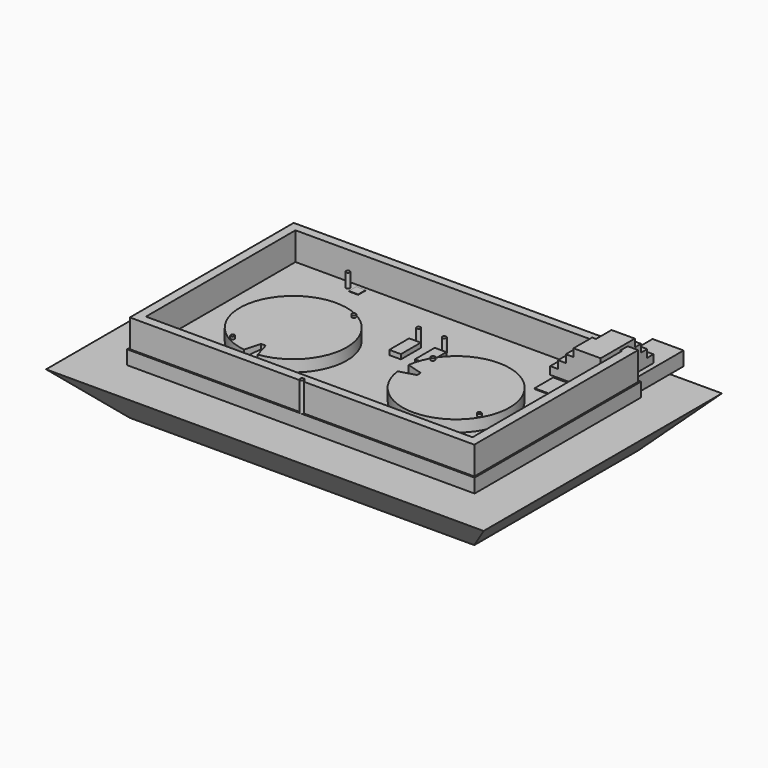
from build123d import *

# Parameters (mm, degrees)
F0_W        = 11277.6
F0_H        = 6705.6
F1_DEPTH    = 457.2
F2_W        = 11277.6
F2_H        = 6705.6
F2_W_2      = 10668
F2_H_2      = 6096
F3_DEPTH    = 914.4
F4_R        = 1752.6
F5_DEPTH    = 381
F6_W        = 304.8
F6_H        = 304.8
F7_DEPTH    = 12.7
F8_W        = 381
F8_H        = 812.8
F9_DEPTH    = 152.4
F11_W       = 11277.6
F11_H       = 6705.6
F12_DEPTH   = 1524
F12_TAPER   = -45
F14_R       = 63.5
F15_DEPTH   = 457.2
F16_DEPTH   = 508
F17_W       = 10693.4
F17_H       = 6121.4
F17_W_2     = 10668
F17_H_2     = 6096
F18_DEPTH   = 914.4
F21_DEPTH   = 228.6
F22_SIZE2   = 533.39999
F22_SIZE    = 76.19999
F22_2_SIZE2 = 533.39999
F22_2_SIZE  = 76.19999
F23_W       = 11379.2
F23_H       = 6807.2
F23_W_2     = 11277.6
F23_H_2     = 6705.6
F24_DEPTH   = 457.2
F25_W       = 1016
F25_H       = 457.2
F26_DEPTH   = 2032
F27_R       = 25.4
F28_DEPTH   = 1816.1010001
F30_DEPTH   = 1016
F32_DEPTH   = 762
F34_DEPTH   = 762
F36_DEPTH   = 25.4


# Not quite as in the source:
# - a fillet or chamfer is up to 0.001 mm smaller than in the source, because OpenCascade refuses the exact size


with BuildPart() as f1:
    # F0 (on Top) → F1 (new body)
    with BuildSketch(Plane.XY):
        Rectangle(F0_W, F0_H)
    extrude(amount=-F1_DEPTH)

    # F23 (on Top) → F24 (join, through all)
    with BuildSketch(Plane.XY):
        Rectangle(F23_W, F23_H)
        Rectangle(F23_W_2, F23_H_2, mode=Mode.SUBTRACT)
    extrude(amount=-F24_DEPTH)

    # F25 (on face) → F26 (join)
    with BuildSketch(Plane(origin=(0, 3403.6, 0), x_dir=(-1, 0, 0), z_dir=(0, 1, 0))):
        with Locations((-4953, -228.6)):
            Rectangle(F25_W, F25_H)
    extrude(amount=F26_DEPTH)

    # F35 (on face) → F36 (join)
    with BuildSketch(Plane.XY):
        with BuildLine():
            Line((5041.9, 2146.3), (3822.7, 2146.3))
            Line((3822.7, 2146.3), (3822.7, 1384.3))
            Line((3822.7, 1384.3), (5041.9, 1384.3))
            Line((5041.9, 1384.3), (5041.9, 1651))
            ThreePointArc((5041.9, 1651), (4927.6, 1765.3), (5041.9, 1879.6))
            Line((5041.9, 1879.6), (5041.9, 2146.3))
        make_face()
        with BuildLine():
            ThreePointArc((5156.2, 1765.3), (5122.7223050896, 1846.1223050896), (5041.9, 1879.6))
            Line((5041.9, 1879.6), (5041.9, 1651))
            ThreePointArc((5041.9, 1651), (5122.7223050896, 1684.4776949104), (5156.2, 1765.3))
        make_face()
        with BuildLine():
            Line((5041.9, 1651), (5041.9, 1879.6))
            ThreePointArc((5041.9, 1879.6), (4927.6, 1765.3), (5041.9, 1651))
        make_face()
    extrude(amount=F36_DEPTH)


with BuildPart() as f3:
    # F2 (on face) → F3 (new body)
    with BuildSketch(Plane.XY):
        Rectangle(F2_W, F2_H)
        Rectangle(F2_W_2, F2_H_2, mode=Mode.SUBTRACT)
    extrude(amount=F3_DEPTH)

    # F17 (on face) → F18 (cut, through all)
    with BuildSketch(Plane.XY.offset(914.4)):
        Rectangle(F17_W, F17_H)
        Rectangle(F17_W_2, F17_H_2, mode=Mode.SUBTRACT)
    extrude(amount=-F18_DEPTH, mode=Mode.SUBTRACT)

    # F27 (on face) → F28 (cut, through all)
    with BuildSketch(Plane.YZ.offset(-5346.7)):
        with Locations((-2984.5, 28.575)):
            Circle(F27_R)
    extrude(amount=-F28_DEPTH, mode=Mode.SUBTRACT)


with BuildPart() as f5:
    # F4 (on face) → F5 (new body)
    with BuildSketch(Plane.XY):
        with Locations((-2667, -381)):
            Circle(F4_R)
    extrude(amount=F5_DEPTH)


with BuildPart() as f5b:
    # F4 (on face) → F5, piece 2 (new body)
    with BuildSketch(Plane.XY):
        with Locations((2667, -381)):
            Circle(F4_R)
    extrude(amount=F5_DEPTH)


with BuildPart() as f7:
    # F6 (on face) → F7 (new body)
    with BuildSketch(Plane.XY):
        with Locations((-3111.5, 2794)):
            Rectangle(F6_W, F6_H)
    extrude(amount=F7_DEPTH)


with BuildPart() as f7b:
    # F6 (on face) → F7, piece 2 (new body)
    with BuildSketch(Plane.XY):
        with Locations((-3111.5, 1524)):
            Rectangle(F6_W, F6_H)
    extrude(amount=F7_DEPTH)


with BuildPart() as f9:
    # F8 (on face) → F9 (new body)
    with BuildSketch(Plane.XY):
        with Locations((-63.5, 939.8)):
            Rectangle(F8_W, F8_H)
    extrude(amount=F9_DEPTH)


with BuildPart() as f9b:
    # F8 (on face) → F9, piece 2 (new body)
    with BuildSketch(Plane.XY):
        with Locations((774.7, 939.8)):
            Rectangle(F8_W, F8_H)
    extrude(amount=F9_DEPTH)


with BuildPart() as f12:
    # F11 (on offset) → F12 (new body)
    with BuildSketch(Plane(origin=(0, 0, -1981.2), x_dir=(1, 0, 0), z_dir=(0, 0, -1))):
        Rectangle(F11_W, F11_H)
    extrude(amount=-F12_DEPTH, taper=F12_TAPER)


with BuildPart() as f15:
    # F14 (on face) → F15 (new body)
    with BuildSketch(Plane.XY):
        with Locations((-63.5, 1498.6)):
            Circle(F14_R)
    extrude(amount=F15_DEPTH)


with BuildPart() as f15b:
    # F14 (on face) → F15, piece 2 (new body)
    with BuildSketch(Plane.XY):
        with Locations((774.7, 1498.6)):
            Circle(F14_R)
    extrude(amount=F15_DEPTH)


with BuildPart() as f15c:
    # F14 (on face) → F15, piece 3 (new body)
    with BuildSketch(Plane.XY):
        with Locations((4097.2159486254, -1220.8497000298)):
            Circle(F14_R)
    extrude(amount=F15_DEPTH)


with BuildPart() as f15d:
    # F14 (on face) → F15, piece 4 (new body)
    with BuildSketch(Plane.XY):
        with Locations((-3416.3, 2794)):
            Circle(F14_R)
    extrude(amount=F15_DEPTH)


with BuildPart() as f15e:
    # F14 (on face) → F15, piece 5 (new body)
    with BuildSketch(Plane.XY):
        with Locations((0, -3352.8)):
            Circle(F14_R)
    extrude(amount=F15_DEPTH)

    # F16 (add): a face of the model
    f16_faces = [f15e.faces().sort_by_distance(p)[0] for p in [
        (0, -3352.8, 457.2),
    ]]
    extrude(f16_faces, amount=F16_DEPTH)


with BuildPart() as f15f:
    # F14 (on face) → F15, piece 6 (new body)
    with BuildSketch(Plane.XY):
        with Locations((1236.7840513746, 458.8497000298)):
            Circle(F14_R)
    extrude(amount=F15_DEPTH)


with BuildPart() as f15g:
    # F14 (on face) → F15, piece 7 (new body)
    with BuildSketch(Plane.XY):
        with Locations((-3506.8497000298, -1811.2159486254)):
            Circle(F14_R)
    extrude(amount=F15_DEPTH)


with BuildPart() as f15h:
    # F14 (on face) → F15, piece 8 (new body)
    with BuildSketch(Plane.XY):
        with Locations((-1827.1502999702, 1049.2159486254)):
            Circle(F14_R)
    extrude(amount=F15_DEPTH)


with BuildPart() as f21_tool:
    # F20 (on face) → F21 (new body)
    with BuildSketch(Plane.XY.offset(381)):
        Polygon((-2743.2, -1600.2), (-2895.6, -2133.6), (-2438.4, -2133.6), (-2590.8, -1600.2), align=None)
        Polygon((1447.8, -304.8), (914.4, -152.4), (914.4, -609.6), (1447.8, -457.2), align=None)
    extrude(amount=-F21_DEPTH)


with BuildPart() as f5_1:
    add(f5.part)

    # F21: cut by f21_tool
    add(f21_tool.part, mode=Mode.SUBTRACT)

    # F22 (size 76.2 and 533.4 in the source; OpenCascade refuses exactly that, so slightly less here)
    f22_edges = [f5_1.edges().sort_by_distance(p)[0] for p in [
        (-2667, -1600.2, 152.4),
    ]]
    chamfer(f22_edges, length=F22_SIZE, length2=F22_SIZE2)


with BuildPart() as f5b_1:
    add(f5b.part)

    # F21: cut by f21_tool
    add(f21_tool.part, mode=Mode.SUBTRACT)

    # F22#2 (size 76.2 and 533.4 in the source; OpenCascade refuses exactly that, so slightly less here)
    f22_2_edges = [f5b_1.edges().sort_by_distance(p)[0] for p in [
        (1447.8, -381, 152.4),
    ]]
    chamfer(f22_2_edges, length=F22_2_SIZE, length2=F22_2_SIZE2)


with BuildPart() as f30:
    # F29 (on face) → F30 (new body)
    with BuildSketch(Plane.XY):
        Polygon((3644.9, 3009.9), (3644.9, 2247.9), (5295.9, 2247.9), (5295.9, 4406.9), (4533.9, 4406.9), (4533.9, 3009.9), align=None)
    extrude(amount=F30_DEPTH)

    # F31 (on face) → F32 (cut)
    with BuildSketch(Plane.YZ.offset(5295.9)):
        Polygon((4152.9, 254), (4406.9, 254), (4406.9, 1016), (3644.9, 1016), (3644.9, 762), (3898.9, 762), (3898.9, 508), (4152.9, 508), align=None)
    extrude(amount=-F32_DEPTH, mode=Mode.SUBTRACT)

    # F33 (on face) → F34 (cut)
    with BuildSketch(Plane(origin=(0, 3009.9, 0), x_dir=(-1, 0, 0), z_dir=(0, 1, 0))):
        Polygon((-3898.9, 254), (-3644.9, 254), (-3644.9, 1016), (-4406.9, 1016), (-4406.9, 762), (-4152.9, 762), (-4152.9, 508), (-3898.9, 508), align=None)
    extrude(amount=-F34_DEPTH, mode=Mode.SUBTRACT)


solid = Compound([f1.part, f3.part, f7.part, f7b.part, f9.part, f9b.part, f12.part, f15.part, f15b.part, f15c.part, f15d.part, f15e.part, f15f.part, f15g.part, f15h.part, f5_1.part, f5b_1.part, f30.part])
